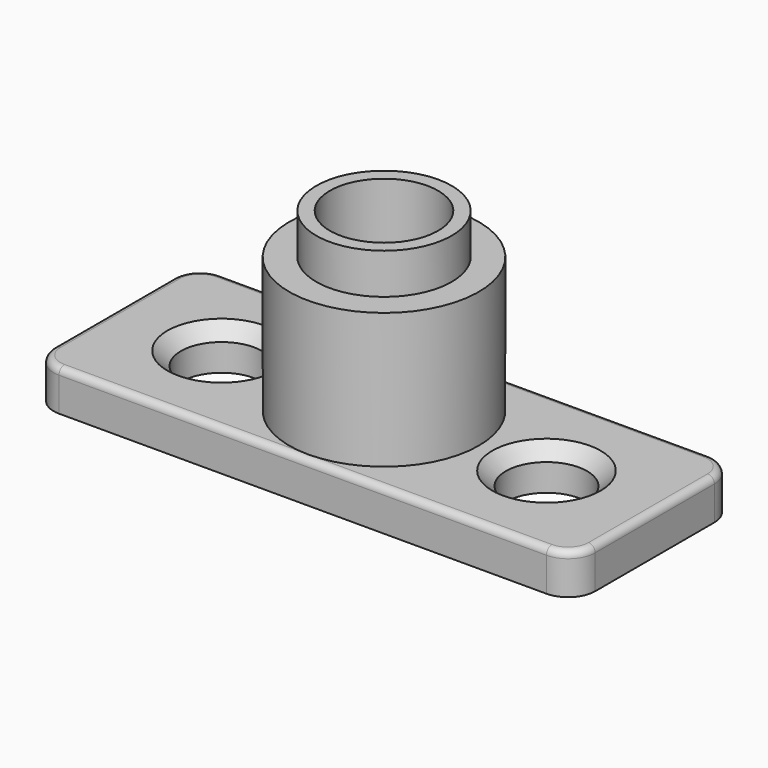
from build123d import *
from build123d import SkipClean  # not in build123d's __all__

# Parameters (mm, degrees)
F0_W           = 20
F0_H           = 15
F1_DEPTH       = 3
F3_DEPTH       = 10
F5_DEPTH       = 3
F7_DEPTH       = 25
F9_D           = 6
F9_CSINK_D     = 8
F9_CSINK_ANGLE = 90
F10_R          = 2
F12_R          = 0.5


with BuildPart() as f1:
    # F0 (on Top) → F1 (new body)
    with BuildSketch(Plane.XY):
        with Locations((-10, 7.5)):
            Rectangle(F0_W, F0_H)
    extrude(amount=F1_DEPTH)

    # F2 (on face) → F3 (join)
    with BuildSketch(Plane.XY.offset(3)):
        with BuildLine():
            Line((0, 0.5), (0, 14.5))
            ThreePointArc((0, 14.5), (-7, 7.5), (0, 0.5))
        make_face()
    extrude(amount=F3_DEPTH)

    # F4 (on face) → F5 (join)
    with BuildSketch(Plane.XY.offset(13)):
        with BuildLine():
            Line((0, 2.5), (0, 12.5))
            ThreePointArc((0, 12.5), (-5, 7.5), (0, 2.5))
        make_face()
    extrude(amount=F5_DEPTH)

    # F6 (on face) → F7 (cut)
    with BuildSketch(Plane.XY.offset(16)):
        with BuildLine():
            Line((0, 3.5), (0, 11.5))
            ThreePointArc((0, 11.5), (-4, 7.5), (0, 3.5))
        make_face()
    extrude(amount=-F7_DEPTH, mode=Mode.SUBTRACT)

    # F9 (through all)
    with Locations(Plane.XY.offset(3)):
        with Locations((-12, 7.5)):
            CounterSinkHole(F9_D / 2, F9_CSINK_D / 2, counter_sink_angle=F9_CSINK_ANGLE)

    # F10
    f10_edges = [f1.edges().sort_by_distance(p)[0] for p in [
        (-20, 0, 1.5),
        (-20, 15, 1.5),
    ]]
    fillet(f10_edges, radius=F10_R)

    # F11: F1 across plane


with BuildPart() as f1_1:
    add(f1.part, clean=False)
    with SkipClean():  # cleaning this boolean's faces spoils the solid; the shape is the same uncleaned
        add(f1.part.mirror(Plane.YZ), clean=False)

    # F12
    f12_edges = [f1_1.edges().sort_by_distance(p)[0] for p in [
        (-9, 0, 3),
        (9, 0, 3),
    ]]
    fillet(f12_edges, radius=F12_R)


solid = f1_1.part
